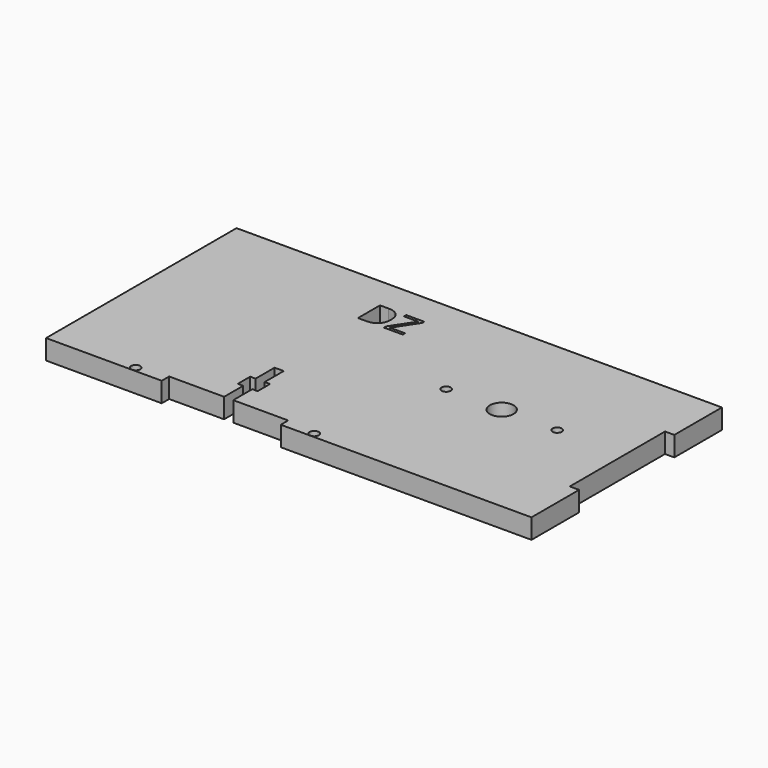
from build123d import *

# Parameters (mm, degrees)
F0_R     = 1.4605
F0_R_2   = 3.81
F1_DEPTH = 6.35


# Not quite as in the source:
# - a feature names something its author has since deleted; it is built from what else it names


with BuildPart() as f1:
    # F0 (on Top) → F1 (new body)
    with BuildSketch(Plane.XY):
        Polygon((72.9530500723, 9.1334713354), (72.9530500723, 28.1834713354), (-82.4187499277, 28.1834713354), (-82.4187499277, -48.0165286646), (-45.3947193277, -48.0165286646), (-45.3947193277, -45.0447286646), (-27.8052193277, -45.0447286646), (-27.8052193277, -37.4247286646), (-29.5197193277, -37.4247286646), (-29.5197193277, -32.4717286646), (-27.8052193277, -32.4717286646), (-27.8052193277, -24.8517286646), (-26.3447193277, -24.8517286646), (-24.8842193277, -24.8517286646), (-24.8842193277, -32.4717286646), (-23.1697193277, -32.4717286646), (-23.1697193277, -37.4247286646), (-24.8842193277, -37.4247286646), (-24.8842193277, -45.0447286646), (-7.2947193277, -45.0447286646), (-7.2947193277, -48.0165286646), (11.7552806723, -48.0165286646), (72.9530500723, -48.0165286646), (72.9530500723, -28.9665286646), (69.9812500723, -28.9665286646), (69.9812500723, 9.1334713354), align=None)
        with Locations((-54.9197193277, -46.5306286646)):
            Circle(F0_R, mode=Mode.SUBTRACT)
        with Locations((2.2302806723, -46.5306286646)):
            Circle(F0_R, mode=Mode.SUBTRACT)
        with BuildLine():
            add(Edge.make_bspline(
                [(-22.4210550397, 16.7985652577), (-21.283380549, 15.660890767), (-21.283380549, 13.6186639082)],
                knots=[0, 0, 0, 1, 1, 1], degree=2))
            add(Edge.make_bspline(
                [(-21.283380549, 13.6186639082), (-21.283380549, 11.4396463825), (-22.4663308238, 10.2865588589)],
                knots=[0, 0, 0, 1, 1, 1], degree=2))
            add(Edge.make_bspline(
                [(-22.4663308238, 10.2865588589), (-23.6492810986, 9.1334713354), (-25.8706844648, 9.1334713354)],
                knots=[0, 0, 0, 1, 1, 1], degree=2))
            Line((-25.8706844648, 9.1334713354), (-28.3097969206, 9.1334713354))
            Line((-28.3097969206, 9.1334713354), (-28.3097969206, 17.9362397483))
            Line((-28.3097969206, 17.9362397483), (-25.6125161638, 17.9362397483))
            add(Edge.make_bspline(
                [(-25.6125161638, 17.9362397483), (-23.5587295303, 17.9362397483), (-22.4210550397, 16.7985652577)],
                knots=[0, 0, 0, 1, 1, 1], degree=2))
        make_face(mode=Mode.SUBTRACT)
        Polygon((-13.9853094725, 10.0601799383), (-13.9853094725, 9.1334713354), (-20.0368515135, 9.1334713354), (-20.0368515135, 9.934949046), (-15.3647759168, 17.0153110328), (-19.8923543301, 17.0153110328), (-19.8923543301, 17.9362397483), (-14.1182468813, 17.9362397483), (-14.1182468813, 17.1347620377), (-18.790322478, 10.0601799383), align=None, mode=Mode.SUBTRACT)
        with Locations((12.9314999741, -7.1371421218)):
            Circle(F0_R, mode=Mode.SUBTRACT)
        with Locations((30.7114999741, -7.1371421218)):
            Circle(F0_R_2, mode=Mode.SUBTRACT)
        with Locations((48.4914999741, -7.1371421218)):
            Circle(F0_R, mode=Mode.SUBTRACT)
    extrude(amount=F1_DEPTH)


solid = f1.part
